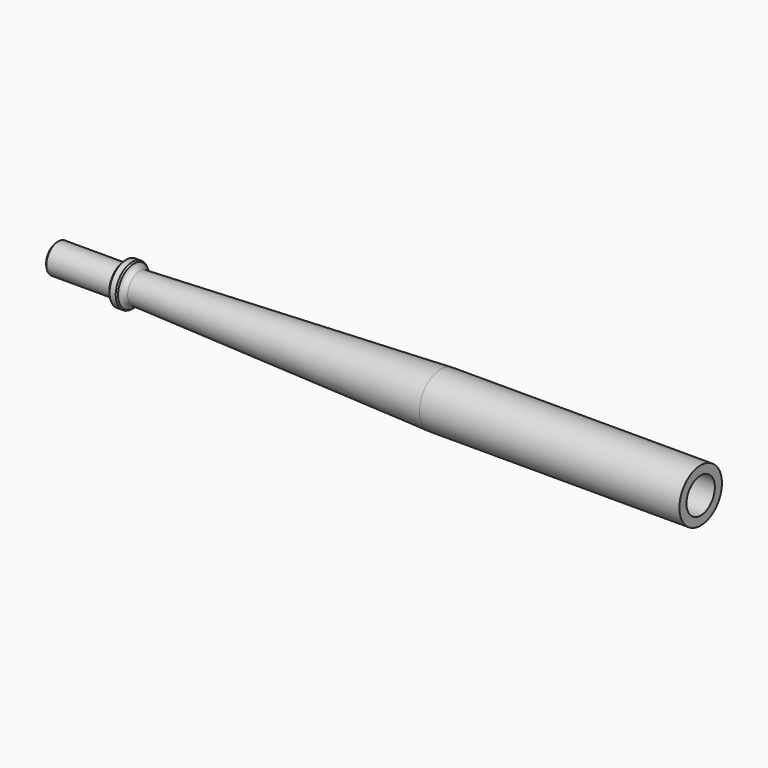
from build123d import *

# Parameters (mm, degrees)
F5_START = 118
F4_R     = 6
F5_DEPTH = 102


# Not quite as in the source:
# - a fillet or chamfer that OpenCascade refuses, or shapes differently, is made with other operations: its cross-section is extruded or revolved along the edge and cut away or added


with BuildPart() as f1:
    # F0 (on Front) → F1 (revolve)
    with BuildSketch(Plane.XZ):
        Polygon((0, 5), (0, 0), (218, 0), (218, 9), (130, 9), (26, 5), (26, 7), (23, 7), (23, 5), align=None)
    revolve(axis=Axis((109, 0, 0), (-1, 0, 0)))

    # F2: fillet of radius 2 on 1 edges, made by hand

    # F2_s1 → F2_t2 (revolve)
    with BuildSketch(Plane.XZ):
        with BuildLine():
            ThreePointArc((28.0753312573, 5.079820433), (26.6401911638, 5.6103195704), (26, 7))
            Line((26, 7), (26, 5))
            Line((26, 5), (28.0753312573, 5.079820433))
        make_face()
    revolve(axis=Axis((26, 0, 0), (-1, 0, 0)))

    # F3: chamfer of 0.5 on 3 edges, made by hand

    # F3_s1 → F3_t2 (revolve, cut)
    with BuildSketch(Plane.XZ):
        Polygon((23, 6.5), (23.5, 7), (23, 7), align=None)
    revolve(axis=Axis((23, 0, 0), (-1, 0, 0)), mode=Mode.SUBTRACT)

    # F3_s3 → F3_t4 (revolve, cut)
    with BuildSketch(Plane.XZ):
        Polygon((0, 4.5), (0.5, 5), (0, 5), align=None)
    revolve(axis=Axis((0, 0, 0), (-1, 0, 0)), mode=Mode.SUBTRACT)

    # F3_s5 → F3_t6 (revolve, cut)
    with BuildSketch(Plane.XZ):
        with BuildLine():
            Line((25.5662808863, 7), (26.0527177117, 6.6156685564))
            ThreePointArc((26.0527177117, 6.6156685564), (26.0180191961, 6.799354671), (26, 7))
            Line((26, 7), (25.5662808863, 7))
        make_face()
    revolve(axis=Axis((26, 0, 0), (-1, 0, 0)), mode=Mode.SUBTRACT)

    # F4 (on Right) → F5 (cut)
    with BuildSketch(Plane.YZ.offset(F5_START)):
        Circle(F4_R)
    extrude(amount=F5_DEPTH, mode=Mode.SUBTRACT)


solid = f1.part
